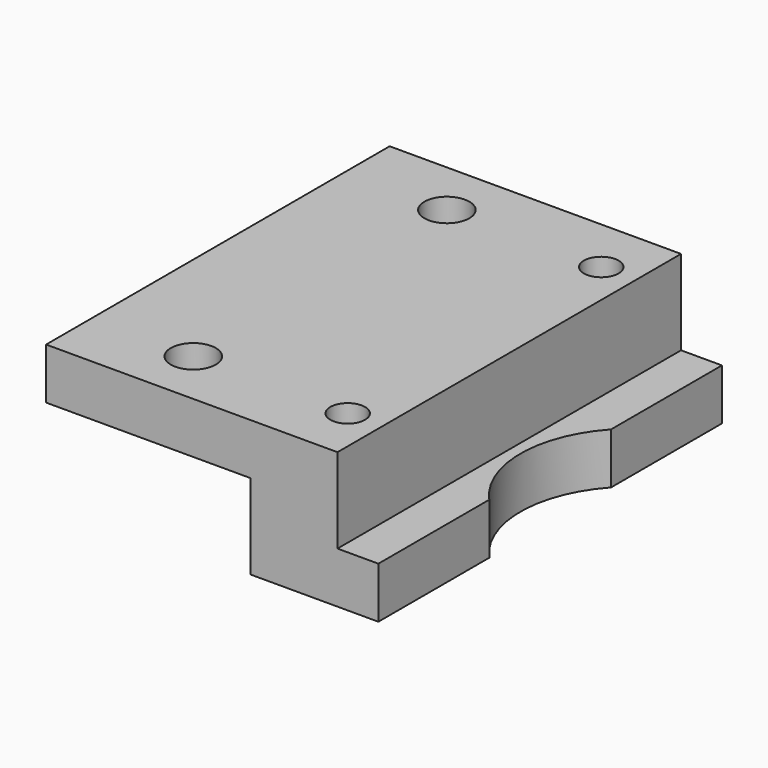
from build123d import *

# Parameters (mm, degrees)
F1_DEPTH     = 42
F2_R         = 1.7
F2_R_2       = 11
F3_DEPTH     = 13.301
F4_W         = 42
F4_H         = 5
F5_DEPTH     = 20
F6_R         = 2.2
F7_DEPTH     = 25
F8_TEXT_SIZE = 39.5833333333
F9_DEPTH     = 1
F10_DEPTH    = 1


# Not quite as in the source:
# - Text() gives the source's letters only with a copy of the font that has no kerning and outlines rounded to 1/6400 em; it was checked with that copy


with BuildPart() as f1:
    # F0 (on Front) → F1 (new body)
    with BuildSketch(Plane.XZ):
        Polygon((8.5, 5), (8.5, 13.3), (0, 13.3), (0, 0), (12.5, 0), (12.5, 5), align=None)
    extrude(amount=-F1_DEPTH)

    # F2 (on face) → F3 (cut, through all)
    with BuildSketch(Plane(origin=(0, 0, 0), x_dir=(1, 0, 0), z_dir=(0, 0, -1))):
        with Locations((5.1, -5.5)):
            Circle(F2_R)
        with Locations((5.1, -36.5)):
            Circle(F2_R)
        with Locations((20.6, -21)):
            Circle(F2_R_2)
    extrude(amount=-F3_DEPTH, mode=Mode.SUBTRACT)

    # F4 (on face) → F5 (join)
    with BuildSketch(Plane(origin=(0, 0, 0), x_dir=(0, -1, 0), z_dir=(-1, 0, 0))):
        with Locations((-21, 10.8)):
            Rectangle(F4_W, F4_H)
    extrude(amount=F5_DEPTH)

    # F6 (on face) → F7 (cut)
    with BuildSketch(Plane.XY.offset(13.3)):
        with Locations((-10, 36.5)):
            Circle(F6_R)
        with Locations((-10, 5.5)):
            Circle(F6_R)
    extrude(amount=-F7_DEPTH, mode=Mode.SUBTRACT)

    # F8 (on face) → F9 (join)
    with BuildSketch(Plane.XY.offset(13.3)):
        with Locations(Location((-20, 31.5050455729), (0, 0, -90))):
            Text('L', F8_TEXT_SIZE, font='Open Sans', font_style=FontStyle.BOLD, text_align=(TextAlign.LEFT, TextAlign.BOTTOM))
    extrude(amount=F9_DEPTH)

    # F10 (cut): a face of the model
    f10_faces = [f1.faces().sort_by_distance(p)[0] for p in [
        (-8.7942463097, 22.7631024165, 14.3),
    ]]
    extrude(f10_faces, amount=-F10_DEPTH, mode=Mode.SUBTRACT)


solid = f1.part
